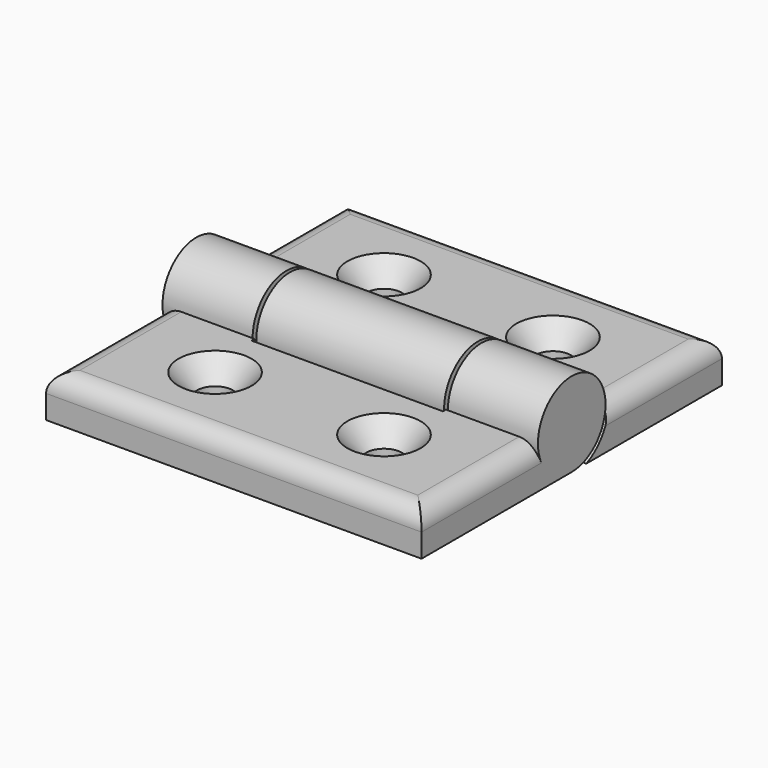
from build123d import *

# Parameters (mm, degrees)
F4_W              = 15.5
F4_H              = 4.5
F7_DEPTH          = 10
F7_DEPTH_BACK     = 10
F8_W              = 0.4
F8_H              = 4.5
F9_DEPTH          = 9.6
F11_DEPTH         = 9.6
F12_DEPTH         = 9.8
F10_W             = 0.4
F10_H             = 4.5
F13_DEPTH         = 9.8
F8_W_2            = 15.1
F14_DEPTH         = 40
F16_DEPTH         = 10
F18_DEPTH         = 10
F19_R             = 2
F19_2_R           = 2
F21_D             = 3.7973
F21_CSINK_D       = 7.7978
F21_CSINK_ANGLE   = 82
F21_2_D           = 3.7973
F21_2_CSINK_D     = 7.7978
F21_2_CSINK_ANGLE = 82


with BuildPart() as f2:
    # F1 (on Front) → F2 (revolve)
    with BuildSketch(Plane.XZ):
        with BuildLine():
            Line((-10, 1.8498126353), (-10, 0))
            Line((-10, 0), (10, 0))
            Line((10, 0), (10, 1.6971506079))
            ThreePointArc((10, 1.6971506079), (-0.0074897347, 0.7922638586), (-10, 1.8498126353))
        make_face()
        with BuildLine():
            Line((-10.4, 0), (-10, 0))
            Line((-10, 0), (-10, 1.8498126353))
            ThreePointArc((-10, 1.8498126353), (-10.2000835145, 1.8914635263), (-10.4, 1.9339088831))
            Line((-10.4, 1.9339088831), (-10.4, 0))
        make_face()
        with BuildLine():
            Line((10, 1.6971506079), (10, 0))
            Line((10, 0), (10.4, 0))
            Line((10.4, 0), (10.4, 1.774885404))
            ThreePointArc((10.4, 1.774885404), (10.2000769588, 1.7356219988), (10, 1.6971506079))
        make_face()
    revolve(axis=Axis((0, 0, 0), (1, 0, 0)))

    # F8 (on offset) → F9 (join, through all)
    with BuildSketch(Plane.YZ.offset(20)):
        with Locations((-4.7, -2.25)):
            Rectangle(F8_W, F8_H)
        with BuildLine():
            ThreePointArc((4.5, 0), (0, 4.5), (-4.5, 0))
            Line((-4.5, 0), (4.5, 0))
        make_face()
        with BuildLine():
            ThreePointArc((0, -4.5), (-3.1819805153, -3.1819805153), (-4.5, 0))
            Line((-4.5, 0), (-4.5, -4.5))
            Line((-4.5, -4.5), (0, -4.5))
        make_face()
        with BuildLine():
            Line((4.5, 0), (-4.5, 0))
            ThreePointArc((-4.5, 0), (-3.1819805153, -3.1819805153), (0, -4.5))
            ThreePointArc((0, -4.5), (3.1819805153, -3.1819805153), (4.5, 0))
        make_face()
    extrude(amount=-F9_DEPTH)

    # F10 (on offset) → F11 (join, through all)
    with BuildSketch(Plane.YZ.offset(-20)):
        with BuildLine():
            ThreePointArc((0, -4.5), (3.1819805153, -3.1819805153), (4.5, 0))
            Line((4.5, 0), (-4.5, 0))
            ThreePointArc((-4.5, 0), (-3.1819805153, -3.1819805153), (0, -4.5))
        make_face()
        with BuildLine():
            Line((-4.5, 0), (4.5, 0))
            ThreePointArc((4.5, 0), (0, 4.5), (-4.5, 0))
        make_face()
        with BuildLine():
            ThreePointArc((0, -4.5), (-3.1819805153, -3.1819805153), (-4.5, 0))
            Line((-4.5, 0), (-4.5, -4.5))
            Line((-4.5, -4.5), (0, -4.5))
        make_face()
    extrude(amount=F11_DEPTH)

    # F8 (on offset) → F12 (join)
    with BuildSketch(Plane.YZ.offset(20)):
        with Locations((-4.7, -2.25)):
            Rectangle(F8_W, F8_H)
    extrude(amount=-F12_DEPTH)

    # F10 (on offset) → F13 (join)
    with BuildSketch(Plane.YZ.offset(-20)):
        with Locations((-4.7, -2.25)):
            Rectangle(F10_W, F10_H)
    extrude(amount=F13_DEPTH)

    # F8 (on offset) → F14 (join, through all)
    with BuildSketch(Plane.YZ.offset(20)):
        with Locations((-12.45, -2.25)):
            Rectangle(F8_W_2, F8_H)
    extrude(amount=-F14_DEPTH)

    # F19
    f19_edges = [f2.edges().sort_by_distance(p)[0] for p in [
        (20, -12.25, 0),
        (0, -20, 0),
        (-20, -12.25, 0),
    ]]
    fillet(f19_edges, radius=F19_R)

    # F21 (through all)
    with Locations(Plane.XY):
        with Locations((9, 11.25), (-9, 11.25), (-9, -11.25), (9, -11.25)):
            CounterSinkHole(F21_D / 2, F21_CSINK_D / 2, counter_sink_angle=F21_CSINK_ANGLE)


with BuildPart() as f3:
    # F1 (on Front) → F3 (revolve)
    with BuildSketch(Plane.XZ):
        with BuildLine():
            Line((-10, 4.5), (-10, 2.2582874036))
            ThreePointArc((-10, 2.2582874036), (-0.0076110898, 1.1922765363), (10, 2.1043815617))
            Line((10, 2.1043815617), (10, 4.5))
            Line((10, 4.5), (-10, 4.5))
        make_face()
    revolve(axis=Axis((0, 0, 0), (1, 0, 0)))

    # F4 (on Right) → F7 (join, two sides)
    with BuildSketch(Plane.YZ) as f7_sk:
        with Locations((12.25, -2.25)):
            Rectangle(F4_W, F4_H)
        with BuildLine():
            Line((4.5, -4.5), (4.5, 0))
            ThreePointArc((4.5, 0), (3.1819805153, -3.1819805153), (0, -4.5))
            Line((0, -4.5), (4.5, -4.5))
        make_face()
    extrude(amount=F7_DEPTH)
    extrude(f7_sk.sketch, amount=-F7_DEPTH_BACK)

    # F15 (on face) → F16 (join, through all)
    with BuildSketch(Plane(origin=(-10, 0, 0), x_dir=(0, -1, 0), z_dir=(-1, 0, 0))):
        with BuildLine():
            ThreePointArc((-1.939071943, -4.5), (-4.0933759002, -2.6933759002), (-4.9, 0))
            Line((-4.9, 0), (-20, 0))
            Line((-20, 0), (-20, -4.5))
            Line((-20, -4.5), (-1.939071943, -4.5))
        make_face()
    extrude(amount=F16_DEPTH)

    # F17 (on face) → F18 (join, through all)
    with BuildSketch(Plane.YZ.offset(10)):
        with BuildLine():
            Line((20, 0), (4.9, 0))
            ThreePointArc((4.9, 0), (4.0933759002, -2.6933759002), (1.939071943, -4.5))
            Line((1.939071943, -4.5), (20, -4.5))
            Line((20, -4.5), (20, 0))
        make_face()
    extrude(amount=F18_DEPTH)

    # F19#2
    f19_2_edges = [f3.edges().sort_by_distance(p)[0] for p in [
        (20, 12.45, 0),
        (0, 20, 0),
        (-20, 12.45, 0),
    ]]
    fillet(f19_2_edges, radius=F19_2_R)

    # F21#2 (through all)
    with Locations(Plane.XY):
        with Locations((9, 11.25), (-9, 11.25), (-9, -11.25), (9, -11.25)):
            CounterSinkHole(F21_2_D / 2, F21_2_CSINK_D / 2, counter_sink_angle=F21_2_CSINK_ANGLE)


solid = Compound([f2.part, f3.part])
